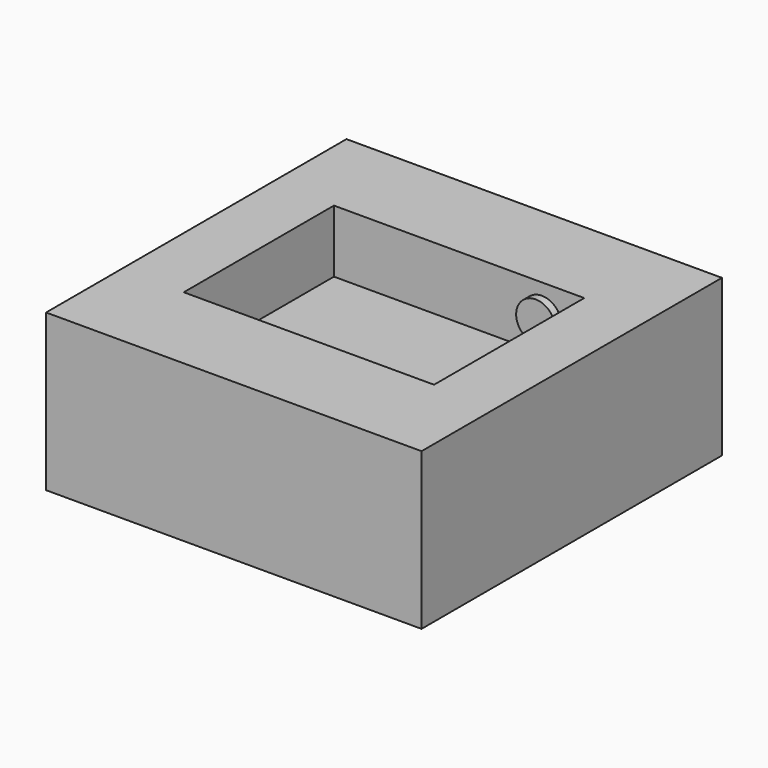
from build123d import *

# Parameters (mm, degrees)
F0_W      = 1200
F0_H      = 1200
F0_W_2    = 1100
F0_H_2    = 1100
F1_DEPTH  = 450
F2_W      = 1200
F2_H      = 1200
F2_W_2    = 1100
F2_H_2    = 1100
F3_DEPTH  = 25
F4_W      = 900
F4_H      = 700
F5_DEPTH  = 200
F6_W      = 1200
F6_H      = 1200
F6_W_2    = 1100
F6_H_2    = 1100
F7_DEPTH  = 25
F8_W      = 800
F8_H      = 600
F9_DEPTH  = 200
F10_R     = 50
F11_DEPTH = 50
F12_R     = 62.5
F12_R_2   = 50
F13_DEPTH = 25


with BuildPart() as f1:
    # F0 (on Top) → F1 (new body)
    with BuildSketch(Plane.XY):
        with Locations((325, 325)):
            Rectangle(F0_W, F0_H)
        with Locations((325, 325)):
            Rectangle(F0_W_2, F0_H_2, mode=Mode.SUBTRACT)
    extrude(amount=F1_DEPTH)

    # F2 (on face) → F3 (join)
    with BuildSketch(Plane.XY.offset(450)):
        with Locations((325, 325)):
            Rectangle(F2_W, F2_H)
        with Locations((325, 325)):
            Rectangle(F2_W_2, F2_H_2, mode=Mode.SUBTRACT)
        with Locations((325, 325)):
            Rectangle(F2_W_2, F2_H_2)
    extrude(amount=F3_DEPTH)

    # F4 (on face) → F5 (join)
    with BuildSketch(Plane(origin=(0, 0, 450), x_dir=(1, 0, 0), z_dir=(0, 0, -1))):
        with Locations((325, -325)):
            Rectangle(F4_W, F4_H)
    extrude(amount=F5_DEPTH)

    # F6 (on face) → F7 (join)
    with BuildSketch(Plane(origin=(0, 0, 0), x_dir=(1, 0, 0), z_dir=(0, 0, -1))):
        with Locations((325, -325)):
            Rectangle(F6_W, F6_H)
        with Locations((325, -325)):
            Rectangle(F6_W_2, F6_H_2, mode=Mode.SUBTRACT)
        with Locations((325, -325)):
            Rectangle(F6_W_2, F6_H_2)
    extrude(amount=F7_DEPTH)

    # F8 (on face) → F9 (cut)
    with BuildSketch(Plane.XY.offset(475)):
        with Locations((325, 325)):
            Rectangle(F8_W, F8_H)
    extrude(amount=-F9_DEPTH, mode=Mode.SUBTRACT)

    # F10 (on face) → F11 (cut, through all)
    with BuildSketch(Plane.XZ.offset(-625)):
        with Locations((589.7976160049, 375)):
            Circle(F10_R)
    extrude(amount=-F11_DEPTH, mode=Mode.SUBTRACT)

    # F12 (on face) → F13 (join)
    with BuildSketch(Plane.XZ.offset(-625)):
        with Locations((589.7976160049, 375)):
            Circle(F12_R)
        with Locations((589.7976160049, 375)):
            Circle(F12_R_2, mode=Mode.SUBTRACT)
        with Locations((589.7976160049, 375)):
            Circle(F12_R_2)
    extrude(amount=F13_DEPTH)


solid = f1.part
